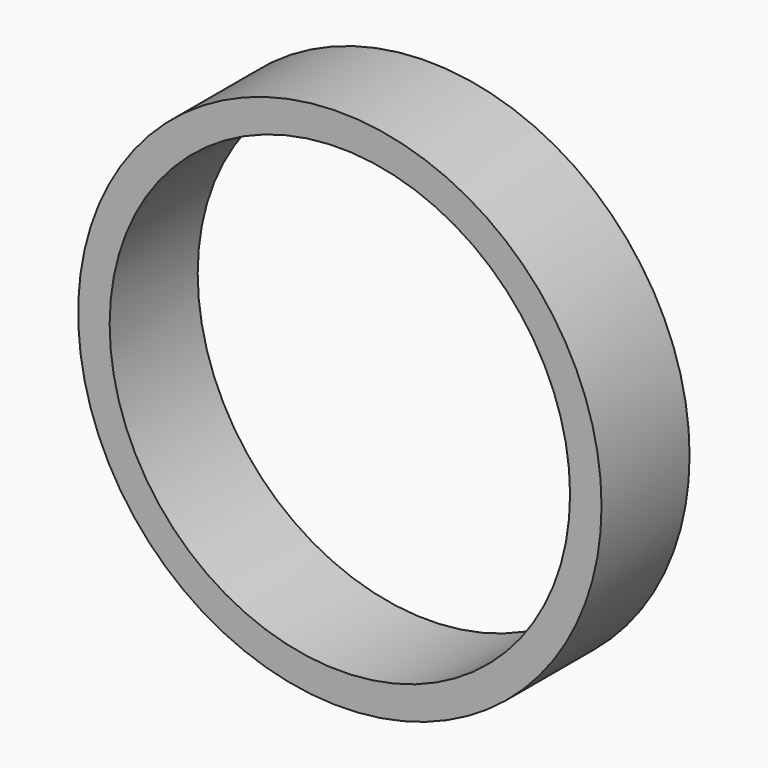
from build123d import *

# Parameters (mm, degrees)
F0_R     = 60.3916892533
F0_R_2   = 53.1274197444
F3_DEPTH = 25.4
F4_DEPTH = 25.4


# Not quite as in the source:
# - the program builds the solid bodies; features that only make, move or delete a surface that nothing else refers to are left out


with BuildPart() as f3:
    # F0 (on Front) → F3 (new body)
    with BuildSketch(Plane.XZ):
        Circle(F0_R)
        Circle(F0_R_2, mode=Mode.SUBTRACT)
    extrude(amount=F3_DEPTH)

    # F0 (on Front) → F4 (join)
    with BuildSketch(Plane.XZ):
        Circle(F0_R)
        Circle(F0_R_2, mode=Mode.SUBTRACT)
    extrude(amount=F4_DEPTH)


solid = f3.part
